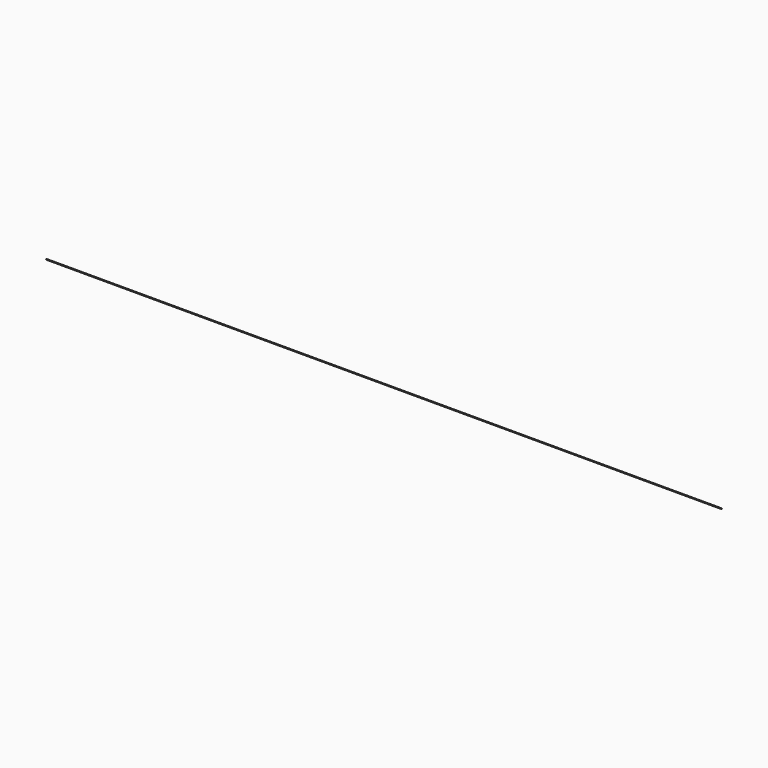
from build123d import *
from build123d import SkipClean  # not in build123d's __all__

# Parameters (mm, degrees)
F2_R     = 0.2286
F3_DEPTH = 436.88


with BuildPart() as f1:
    # F0 (on Top) → F1 (revolve)
    with BuildSketch(Plane.XY):
        with BuildLine():
            Line((0, 0.2286), (0, -0.2286))
            ThreePointArc((0, -0.2286), (0.2286, 0), (0, 0.2286))
        make_face()
    revolve(axis=Axis((0, 0, 0), (0, -1, 0)))

    # F2 (on Right) → F3 (join)
    with BuildSketch(Plane.YZ):
        Circle(F2_R)
    with SkipClean():  # cleaning this boolean's faces spoils the solid; the shape is the same uncleaned
        extrude(amount=-F3_DEPTH)


solid = f1.part
